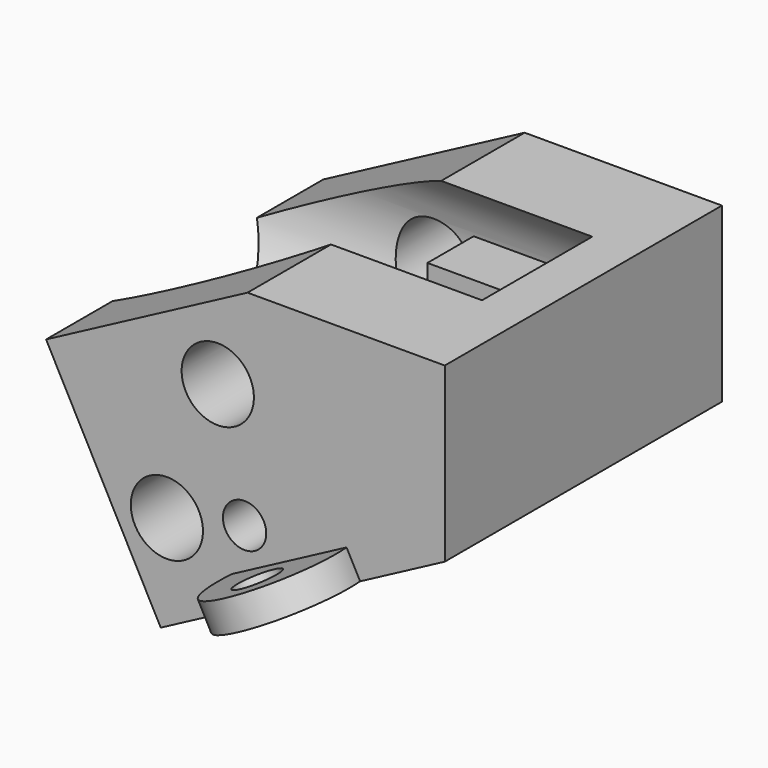
from build123d import *

# Parameters (mm, degrees)
F0_W      = 50.8
F0_H      = 38.1
F1_DEPTH  = 50.8
F3_R      = 10.7442
F4_DEPTH  = 40.64
F5_DEPTH  = 45.72
F7_DEPTH  = 38.101
F9_W      = 6.35
F9_H      = 12.7
F10_DEPTH = 9.525
F11_DEPTH = 38.101
F13_DEPTH = 38.101
F20_R     = 2.38125
F20_R_2   = 3.96875
F20_R_3   = 3.9751
F21_DEPTH = 38.101
F22_DEPTH = 3.175
F23_R     = 2.3876
F24_DEPTH = 3.175


# Not quite as in the source:
# - a feature names something its author has since deleted; it is built from what else it names


with BuildPart() as f1:
    # F0 (on Top) → F1 (new body)
    with BuildSketch(Plane.XY):
        with Locations((25.4, -19.05)):
            Rectangle(F0_W, F0_H)
    extrude(amount=F1_DEPTH)

    # F3 (on face) → F4 (cut)
    with BuildSketch(Plane(origin=(0, 0, 0), x_dir=(0, -1, 0), z_dir=(-1, 0, 0))):
        with Locations((19.05, 43.18)):
            Circle(F3_R)
    extrude(amount=-F4_DEPTH, mode=Mode.SUBTRACT)

    # F3 (on face) → F5 (cut)
    with BuildSketch(Plane(origin=(0, 0, 0), x_dir=(0, -1, 0), z_dir=(-1, 0, 0))):
        with Locations((19.05, 43.18)):
            Circle(F3_R)
    extrude(amount=-F5_DEPTH, mode=Mode.SUBTRACT)

    # F6 (on face) → F7 (cut, through all)
    with BuildSketch(Plane.XZ.offset(38.1)):
        Polygon((-5.2975248545, 32.5760431588), (29.6258907765, 51.0742887855), (29.3069556355, 56.4961917698), (-5.2975248545, 56.4961917698), align=None)
    extrude(amount=-F7_DEPTH, mode=Mode.SUBTRACT)

    # F9 (on face) → F10 (join)
    with BuildSketch(Plane(origin=(45.72, 0, 0), x_dir=(0, -1, 0), z_dir=(-1, 0, 0))):
        with Locations((19.05, 43.18)):
            Rectangle(F9_W, F9_H)
    extrude(amount=F10_DEPTH)

    # F8 (on face) → F11 (cut, through all)
    with BuildSketch(Plane.XZ.offset(38.1)):
        Polygon((12.6081767879, 11.5786670478), (0, 35.3820377673), (-3.8052792661, 35.2523848414), (-3.8052792661, -3.7349041086), (52.9321556466, -3.7349041086), (52.9321556466, 32.9374846805), align=None)
    extrude(amount=-F11_DEPTH, mode=Mode.SUBTRACT)

    # F12 (on face) → F13 (cut, through all)
    with BuildSketch(Plane.XZ.offset(38.1)):
        Polygon((21.0712682456, 12.4185690656), (5.5156808657, 41.7864482914), (-6.4950456949, 35.4714418711), (9.0799157449, 6.0669857527), align=None)
    extrude(amount=-F13_DEPTH, mode=Mode.SUBTRACT)


with BuildPart() as f1_1:
    # F14: moved
    add(f1.part.moved(Location((12.8, 76.1, -11.5))))


with BuildPart() as f1_2:
    # F16: moved
    add(f1_1.part.moved(Location((-7.9, 0, 0))))


with BuildPart() as f1_3:
    # F17: moved
    add(f1_2.part.moved(Location((1.3, 0, -3.7))))


with BuildPart() as f1_4:
    # F18: moved
    add(f1_3.part.moved(Location((0.5, 0, -3.8))))


with BuildPart() as f1_5:
    # F19: moved
    add(f1_4.part.moved(Location((-1.016, 0, 4.064))))

    # F20 (on face) → F21 (cut, through all)
    with BuildSketch(Plane(origin=(0, 76.1, 0), x_dir=(-1, 0, 0), z_dir=(0, 1, 0))):
        with Locations((-34.4707481563, 13.2179586217)):
            Circle(F20_R)
        with Locations((-25.9255170822, 11.1699821427)):
            Circle(F20_R_2)
        with Locations((-31.5185599029, 25.9363166988)):
            Circle(F20_R_3)
    extrude(amount=-F21_DEPTH, mode=Mode.SUBTRACT)

    # F22 (add): a face of the model
    f22_faces = [f1_5.faces().sort_by_distance(p)[0] for p in [
        (40.8662395369, 57.05, 8.5997036085),
    ]]
    extrude(f22_faces, amount=-F22_DEPTH)

    # F23 (on face) → F24 (join)
    with BuildSketch(Plane(origin=(5.3963751445, 0, -10.1879851676), x_dir=(0.8836897656, 0, 0.4680730692), z_dir=(0.4680730692, 0, -0.8836897656))):
        with BuildLine():
            Line((32.9755673007, -38), (47.2757673007, -38))
            ThreePointArc((47.2757673007, -38), (40.1256673007, -29.0169325565), (32.9755673007, -38))
        make_face()
        with Locations((40.1383673007, -33.5931)):
            Circle(F23_R, mode=Mode.SUBTRACT)
        with BuildLine():
            ThreePointArc((32.9755673007, -76.1), (40.1256673007, -85.0830674435), (47.2757673007, -76.1))
            Line((47.2757673007, -76.1), (32.9755673007, -76.1))
        make_face()
        with Locations((40.1383673007, -80.5069)):
            Circle(F23_R, mode=Mode.SUBTRACT)
    extrude(amount=-F24_DEPTH)


solid = f1_5.part
